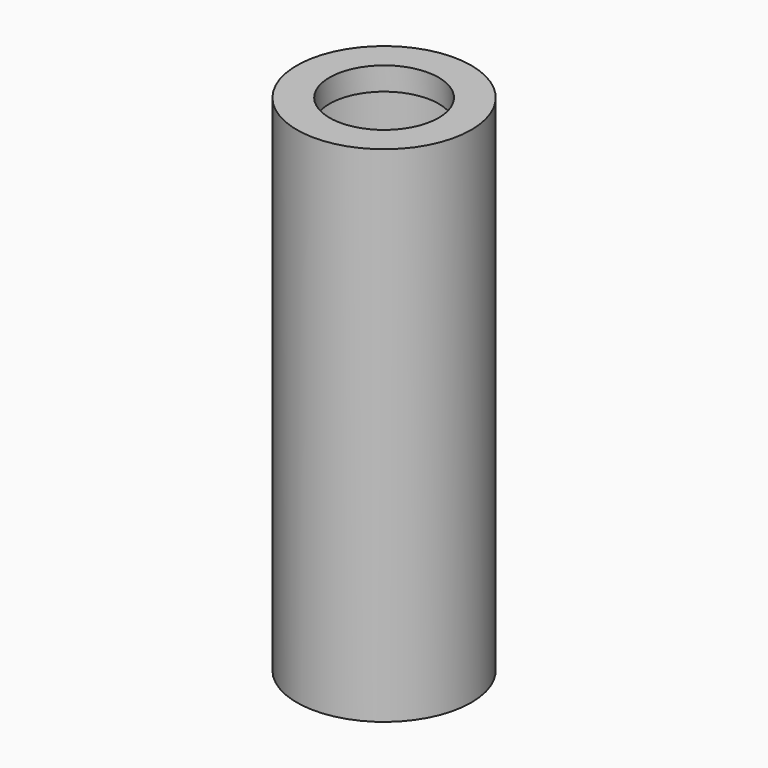
from build123d import *

# Parameters (mm, degrees)
F0_R     = 15.4
F0_R_2   = 14.65
F1_DEPTH = 89
F2_W     = 5.0115964577
F2_H     = 4.0804579258


# Not quite as in the source:
# - a feature names something its author has since deleted; it is built from what else it names


with BuildPart() as f1:
    # F0 (on Top) → F1 (new body)
    with BuildSketch(Plane.XY):
        Circle(F0_R)
        Circle(F0_R_2, mode=Mode.SUBTRACT)
    extrude(amount=F1_DEPTH)

    # F2 (on Front) → F3 (revolve)
    with BuildSketch(Plane.XZ):
        with Locations((12.1442017712, 86.9597710371)):
            Rectangle(F2_W, F2_H)
    revolve(axis=Axis((0, 0, 68.6147660017), (0, 0, 1)))


solid = f1.part
